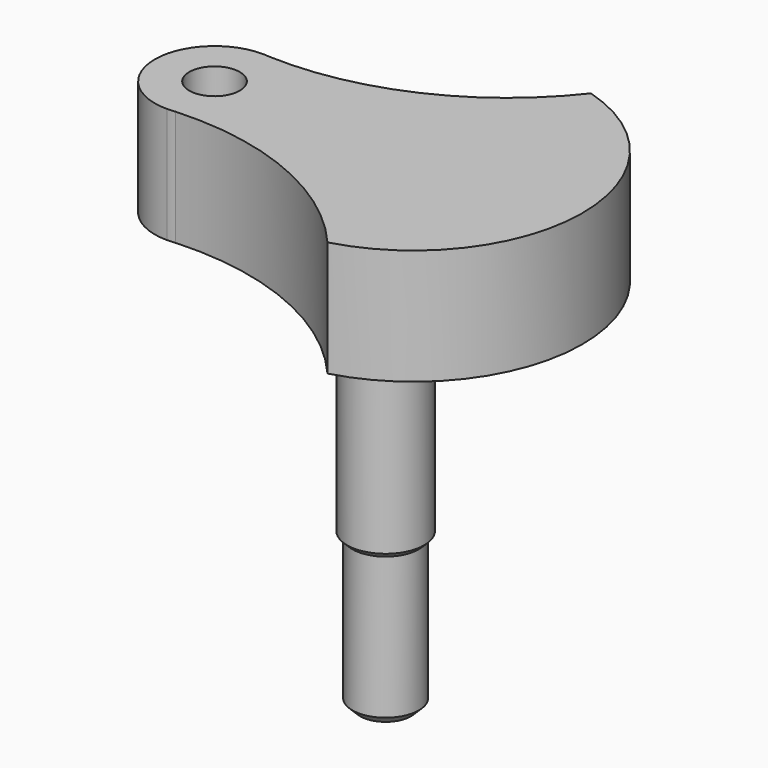
from build123d import *

# Parameters (mm, degrees)
F0_R        = 2.5019
F1_DEPTH    = 11.43
F2_R        = 3.81
F3_DEPTH    = 23.0124
F4_R        = 3.2888740004
F5_DEPTH    = 14.5542
F6_S5_R     = 3.2888740004
F6_T6_DEPTH = 7
F7_SIZE     = 0.762


# Not quite as in the source:
# - a fillet or chamfer that OpenCascade refuses, or shapes differently, is made with other operations: its cross-section is extruded or revolved along the edge and cut away or added


with BuildPart() as f1:
    # F0 (on Top) → F1 (new body)
    with BuildSketch(Plane.XY):
        with BuildLine():
            ThreePointArc((23.9757987458, 16.602474899), (13.6238224038, 8.4064756981), (0.6664771358, 5.8677711678))
            ThreePointArc((0.6664771358, 5.8677711678), (4.4051566928, 3.9331316736), (5.9055, 0))
            ThreePointArc((5.9055, 0), (4.4601151914, -3.8706979641), (0.8314833277, -5.8466713372))
            ThreePointArc((0.8314833277, -5.8466713372), (13.3845311249, -8.052459978), (23.6582204203, -15.5953918211))
            ThreePointArc((23.6582204203, -15.5953918211), (35.9831697874, 0.3835426329), (23.9757987458, 16.602474899))
        make_face()
        with BuildLine():
            ThreePointArc((0.6664771358, 5.8677711678), (0.333126091, 5.8846486866), (0, 5.9055))
            ThreePointArc((0, 5.9055), (-5.9055, 0), (0, -5.9055))
            ThreePointArc((0, -5.9055), (0.4155226631, -5.8729903159), (0.8314833277, -5.8466713372))
            ThreePointArc((0.8314833277, -5.8466713372), (4.4601151914, -3.8706979641), (5.9055, 0))
            ThreePointArc((5.9055, 0), (4.4051566928, 3.9331316736), (0.6664771358, 5.8677711678))
        make_face()
        Circle(F0_R, mode=Mode.SUBTRACT)
        with BuildLine():
            ThreePointArc((0.6664771358, 5.8677711678), (0.3337720919, 5.8960602474), (0, 5.9055))
            ThreePointArc((0, 5.9055), (0.333126091, 5.8846486866), (0.6664771358, 5.8677711678))
        make_face()
        with BuildLine():
            ThreePointArc((0.8314833277, -5.8466713372), (0.4155226631, -5.8729903159), (0, -5.9055))
            ThreePointArc((0, -5.9055), (0.4167809184, -5.8907744751), (0.8314833277, -5.8466713372))
        make_face()
    extrude(amount=F1_DEPTH)

    # F2 (on face) → F3 (join)
    with BuildSketch(Plane(origin=(0, 0, 0), x_dir=(1, 0, 0), z_dir=(0, 0, -1))):
        with Locations((16.9372853817, 0)):
            Circle(F2_R)
    extrude(amount=F3_DEPTH)

    # F4 (on face) → F5 (join)
    with BuildSketch(Plane(origin=(0, 0, -23.0124), x_dir=(1, 0, 0), z_dir=(0, 0, -1))):
        with Locations((16.9372853817, 0)):
            Circle(F4_R)
    extrude(amount=F5_DEPTH)

    # F6: chamfer of 0.762 on 1 edges, made by hand


with BuildPart() as f6_tool2:
    # F6_s3 → F6_t4 (revolve)
    with BuildSketch(Plane.XZ):
        Polygon((20.7472853817, -22.2504), (19.9852853817, -23.0124), (20.7472853817, -23.0124), align=None)
    revolve(axis=Axis((16.9372853817, 0, -23.0124), (0, 0, -1)))

    # F6_s5 → F6_t6 (cut, symmetric)
    with BuildSketch(Plane.XY.offset(-22.6)):
        with Locations((16.9372853817, 0)):
            Circle(F6_S5_R)
    extrude(amount=F6_T6_DEPTH, both=True, mode=Mode.SUBTRACT)


with BuildPart() as f1_1:
    add(f1.part)

    # F6_t1: cut F6_tool2
    add(f6_tool2.part, mode=Mode.SUBTRACT)

    # F7
    f7_edges = [f1_1.edges().sort_by_distance(p)[0] for p in [
        (13.648411, 0, -37.5666),
    ]]
    chamfer(f7_edges, length=F7_SIZE)


solid = f1_1.part
